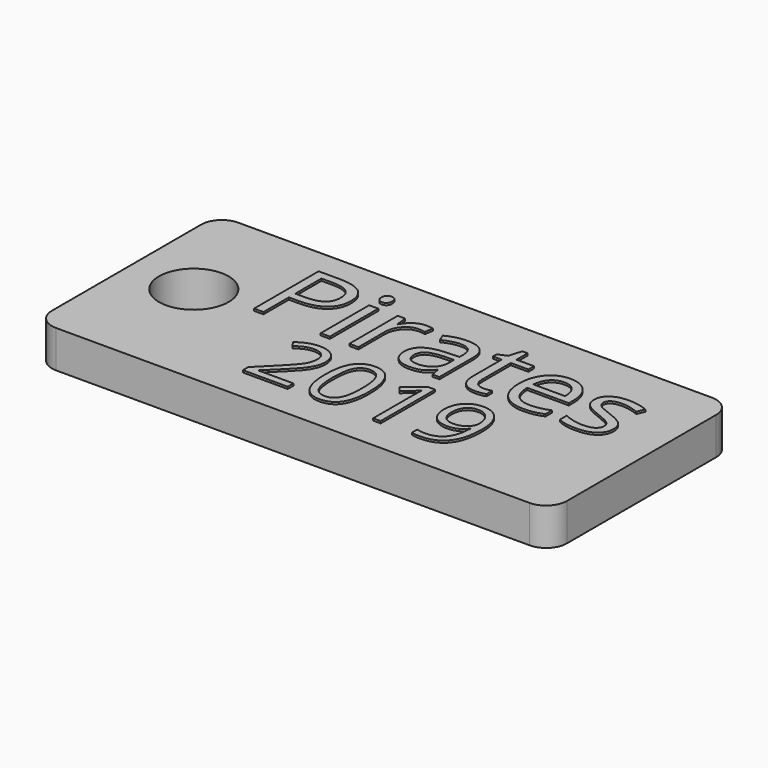
from build123d import *

# Parameters (mm, degrees)
F0_W           = 126.1543817818
F0_H           = 55.84856309
F1_DEPTH       = 9.144
F2_R           = 8.5323838533
F3_DEPTH       = 25.4
F4_R           = 5.08
F5_R           = 5.08
F6_R           = 5.08
F7_R           = 5.08
F8_TEXT_SIZE   = 27.6766641362
F8_TEXT_SIZE_2 = 23.3802601643
F9_DEPTH       = 0.508


# Not quite as in the source:
# - Text() gives the source's letters only with a copy of the font that has no kerning and outlines rounded to 1/6400 em; it was checked with that copy


with BuildPart() as f1:
    # F0 (on Top) → F1 (new body)
    with BuildSketch(Plane.XY):
        with Locations((1.9804444164, 6.0403598472)):
            Rectangle(F0_W, F0_H)
    extrude(amount=F1_DEPTH)

    # F2 (on face) → F3 (cut)
    with BuildSketch(Plane.XY.offset(9.144)):
        with Locations((-45.4776659608, 7.1286368184)):
            Circle(F2_R)
    extrude(amount=-F3_DEPTH, mode=Mode.SUBTRACT)

    # F4
    f4_edges = [f1.edges().sort_by_distance(p)[0] for p in [
        (65.057635, -21.883922, 4.572),
    ]]
    fillet(f4_edges, radius=F4_R)

    # F5
    f5_edges = [f1.edges().sort_by_distance(p)[0] for p in [
        (65.057635, 33.964641, 4.572),
    ]]
    fillet(f5_edges, radius=F5_R)

    # F6
    f6_edges = [f1.edges().sort_by_distance(p)[0] for p in [
        (-61.096746, -21.883922, 4.572),
    ]]
    fillet(f6_edges, radius=F6_R)

    # F7
    f7_edges = [f1.edges().sort_by_distance(p)[0] for p in [
        (-61.096746, 33.964641, 4.572),
    ]]
    fillet(f7_edges, radius=F7_R)

    # F8 (on face) → F9 (join)
    with BuildSketch(Plane.XY.offset(9.144)):
        with Locations((-33.5685536265, 7.3039288457)):
            Text('Pirates', F8_TEXT_SIZE, font='Open Sans', text_align=(TextAlign.LEFT, TextAlign.BOTTOM))
        with Locations((-17.7249865374, -13.9621412382)):
            Text('2019', F8_TEXT_SIZE_2, font='Open Sans', text_align=(TextAlign.LEFT, TextAlign.BOTTOM))
    extrude(amount=F9_DEPTH)


solid = f1.part
